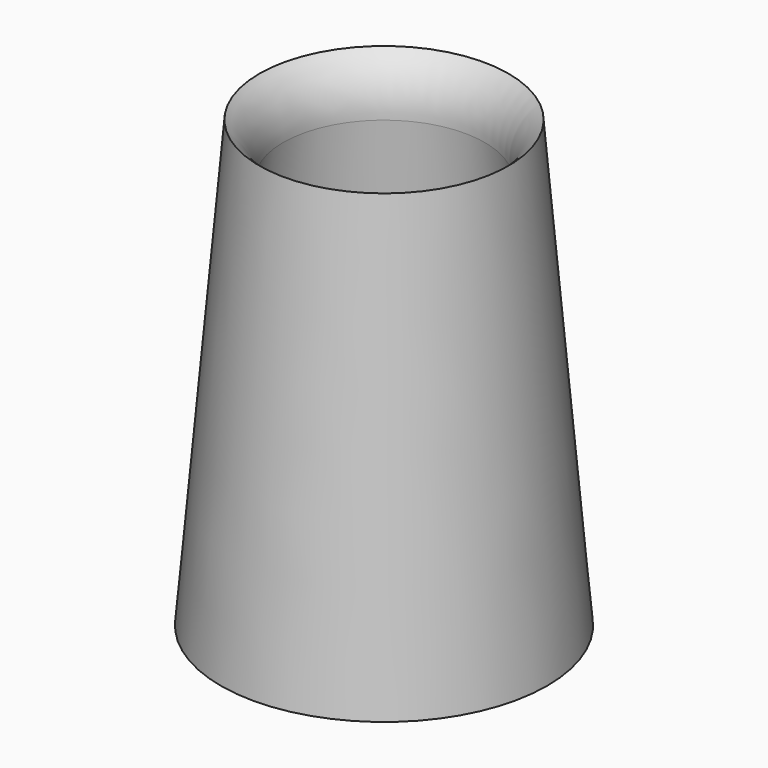
from build123d import *


# Not quite as in the source:
# - a fillet or chamfer that OpenCascade refuses, or shapes differently, is made with other operations: its cross-section is extruded or revolved along the edge and cut away or added


with BuildPart() as f1:
    # F0 (on Front) → F1 (revolve)
    with BuildSketch(Plane.XZ):
        Polygon((-45, 0), (-45, 5), (-44.1333333333, 15), (-32.417820976, 150.1789887381), (-42, 150), (-55, 0), align=None)
        Polygon((-45, 5), (0, 5), (0, 15), (-44.1333333333, 15), align=None)
    revolve(axis=Axis((0, 0, 75), (0, 0, 1)))

    # F2: fillet of radius 20 on 1 edges, made by hand

    # F2_s1 → F2_t2 (revolve, cut)
    with BuildSketch(Plane.XZ):
        with BuildLine():
            ThreePointArc((-33.9760329601, 132.1996196909), (-35.6682042477, 142.1455232835), (-42, 150))
            Line((-42, 150), (-32.417820976, 150.1789887381))
            Line((-32.417820976, 150.1789887381), (-33.9760329601, 132.1996196909))
        make_face()
    revolve(axis=Axis((0, 0, 150.1789887381), (0, 0, 1)), mode=Mode.SUBTRACT)


solid = f1.part
